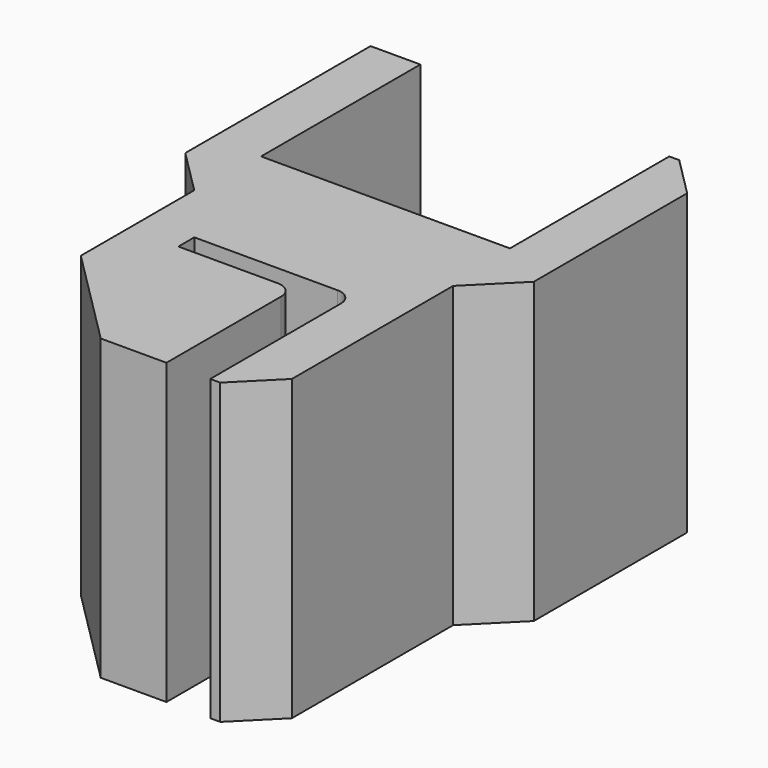
from build123d import *

# Parameters (mm, degrees)
F0_W        = 7.366
F0_H        = 10.16
F1_DEPTH    = 19.05
F2_T4_DEPTH = 19.05
F2_T9_DEPTH = 19.05
F3_SIZE     = 2.54
F4_SIZE     = 6.35
F5_R        = 1.016


# Not quite as in the source:
# - a fillet or chamfer that OpenCascade refuses, or shapes differently, is made with other operations: its cross-section is extruded or revolved along the edge and cut away or added


with BuildPart() as f1:
    # F0 (on Top) → F1 (new body)
    with BuildSketch(Plane.XY):
        Polygon((0, 20.4722661398), (0, 0), (3.175, 0), (3.175, 10.16), (3.175, 11.43), (8.255, 11.43), (13.335, 11.43), (13.335, 0), (16.51, 0), (16.51, 20.4722661398), (19.3675, 20.4722661398), (19.3675, 33.02), (16.1925, 33.02), (16.1925, 20.32), (8.255, 20.32), (0.3175, 20.32), (0.3175, 33.02), (-2.8575, 33.02), (-2.8575, 20.4722661398), align=None)
        with Locations((6.858, 5.08)):
            Rectangle(F0_W, F0_H)
    extrude(amount=F1_DEPTH)

    # F2: chamfer of 5.08 on 2 edges, made by hand


with BuildPart() as f2_tool2:
    # F2_s3 → F2_t4 (new body)
    with BuildSketch(Plane.XY):
        Polygon((-5.08, 20.4722661398), (0, 15.3922661398), (0, 20.4722661398), align=None)
    extrude(amount=F2_T4_DEPTH)

    split(bisect_by=Plane.YZ.offset(-2.8575), keep=Keep.TOP)


with BuildPart() as f1_1:
    add(f1.part)

    # F2_t1: union F2_tool2
    add(f2_tool2.part)


with BuildPart() as f2_tool7:
    # F2_s8 → F2_t9 (new body)
    with BuildSketch(Plane.XY):
        Polygon((16.51, 15.3922661398), (21.59, 20.4722661398), (16.51, 20.4722661398), align=None)
    extrude(amount=F2_T9_DEPTH)

    split(bisect_by=Plane.YZ.offset(19.3675), keep=Keep.BOTTOM)


with BuildPart() as f1_2:
    add(f1_1.part)

    # F2_t6: union F2_tool7
    add(f2_tool7.part)

    # F3
    f3_edges = [f1_2.edges().sort_by_distance(p)[0] for p in [
        (16.51, 0, 9.525),
        (19.3675, 33.02, 9.525),
    ]]
    chamfer(f3_edges, length=F3_SIZE)

    # F4
    f4_edges = [f1_2.edges().sort_by_distance(p)[0] for p in [
        (0, 0, 9.525),
    ]]
    chamfer(f4_edges, length=F4_SIZE)

    # F5
    f5_edges = [f1_2.edges().sort_by_distance(p)[0] for p in [
        (13.335, 11.43, 9.525),
        (10.541, 10.16, 9.525),
    ]]
    fillet(f5_edges, radius=F5_R)


solid = f1_2.part
